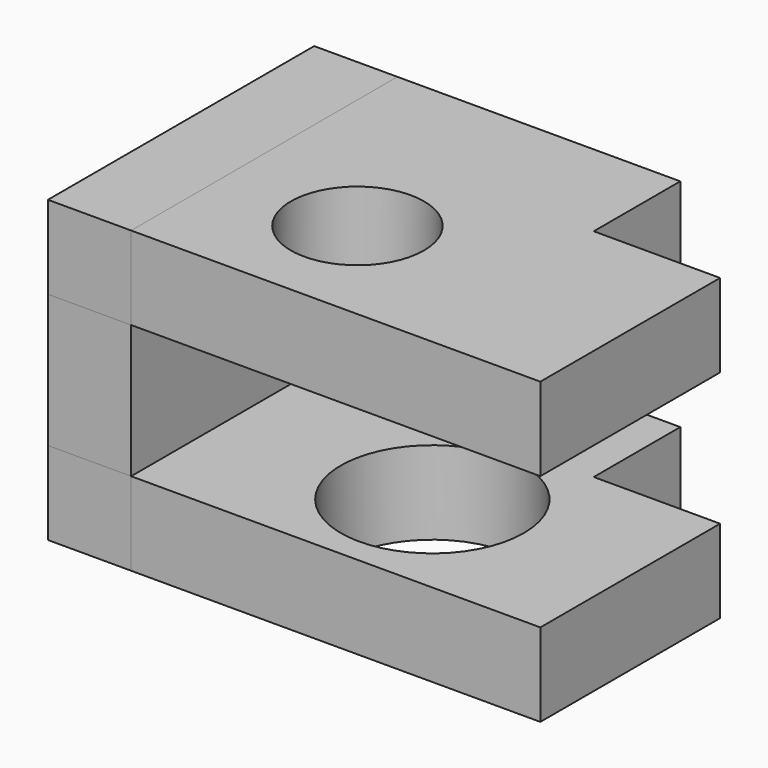
from build123d import *

# Parameters (mm, degrees)
F0_R     = 8
F0_W     = 15.1825966239
F0_H     = 27
F1_DEPTH = 10
F0_W_2   = 10
F0_H_2   = 40
F2_DEPTH = 16
F3_DEPTH = 10
F5_DEPTH = 10
F4_W     = 5
F4_H     = 40.000000447
F4_H_2   = 40
F6_DEPTH = 10


# Not quite as in the source:
# - ends of sketch curves that miss each other by under 0.0002 mm in the source are joined


with BuildPart() as f1:
    # F0 (on Top) → F1 (new body)
    with BuildSketch(Plane.XY):
        Polygon((17, 20), (-17, 20), (-17, -20), (17, -20), (17, 7), align=None)
        with Locations((-1, -6)):
            Circle(F0_R, mode=Mode.SUBTRACT)
        with Locations((24.5912983119, -6.5)):
            Rectangle(F0_W, F0_H)
    extrude(amount=F1_DEPTH)


with BuildPart() as f2:
    # F0 (on Top) → F2 (new body)
    with BuildSketch(Plane.XY):
        with Locations((-22, 0)):
            Rectangle(F0_W_2, F0_H_2)
    extrude(amount=-F2_DEPTH)

    # F4 (on face) → F5 (join)
    with BuildSketch(Plane(origin=(0, 0, -16), x_dir=(1, 0, 0), z_dir=(0, 0, -1))):
        with BuildLine():
            Line((-17, 20.000000447), (-17, -19.999999553))
            Line((-17, -19.999999553), (17, -19.999999553))
            Line((17, -19.999999553), (17, -6.999999553))
            Line((17, -6.999999553), (17, -0.3245548733))
            ThreePointArc((17, -0.3245548733), (-3, 6.000000447), (17, 12.3245557674))
            Line((17, 12.3245557674), (17, 20.000000447))
            Line((17, 20.000000447), (-17, 20.000000447))
        make_face()
        with BuildLine():
            Line((17, -0.3245548733), (17, -6.999999553))
            Line((17, -6.999999553), (32.1825966239, -6.999999553))
            Line((32.1825966239, -6.999999553), (32.1825966239, 20.000000447))
            Line((32.1825966239, 20.000000447), (17, 20.000000447))
            Line((17, 20.000000447), (17, 12.3245557674))
            ThreePointArc((17, 12.3245557674), (18.4880884817, 9.3166252374), (19, 6.000000447))
            ThreePointArc((19, 6.000000447), (18.4880884817, 2.6833756567), (17, -0.3245548733))
        make_face()
    extrude(amount=F5_DEPTH)


with BuildPart() as f3:
    # F0 (on Top) → F3 (new body)
    with BuildSketch(Plane.XY):
        with Locations((-22, 0)):
            Rectangle(F0_W_2, F0_H_2)
    extrude(amount=F3_DEPTH)


with BuildPart() as f6:
    # F4 (on face) → F6 (new body)
    with BuildSketch(Plane(origin=(0, 0, -16), x_dir=(1, 0, 0), z_dir=(0, 0, -1))):
        with Locations((-19.5, 2.235e-07)):
            Rectangle(F4_W, F4_H)
        with Locations((-24.5, 4.47e-07)):
            Rectangle(F4_W, F4_H_2)
    extrude(amount=F6_DEPTH)


solid = Compound([f1.part, f2.part, f3.part, f6.part])
